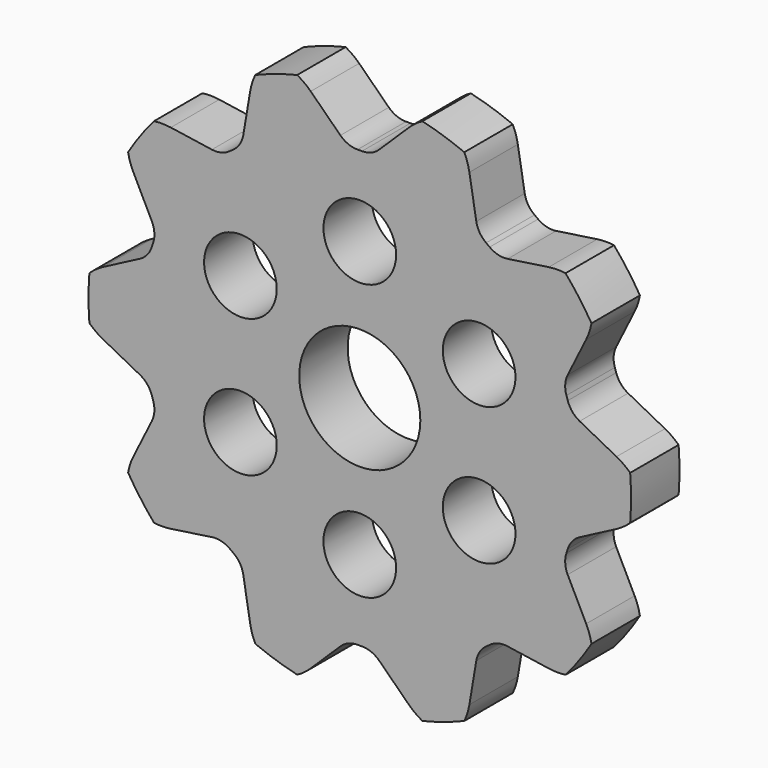
from build123d import *

# Parameters (mm, degrees)
F1_DEPTH        = 25
F3_DEPTH        = 25.001
F3_COPIES_COUNT = 10
F4_R            = 25
F5_DEPTH        = 25.001
F6_R            = 15
F7_DEPTH        = 25.001
F7_COPIES_COUNT = 6


# Not quite as in the source:
# - a pattern or mirror of a feature is missing from the dataset's text; its kind, count and spacing are read off the source's solid


with BuildPart() as f1:
    # F0 (on Front) → F1 (new body)
    with BuildSketch(Plane.XZ):
        with BuildLine():
            Line((-8.9100863455, 98.6570205686), (0, 100))
            Line((0, 100), (13.2558165823, 98.002007127))
            Line((13.2558165823, 98.002007127), (20.2559942473, 104.8591660301))
            ThreePointArc((20.2559942473, 104.8591660301), (22.9030212669, 107.1136465319), (25.8372403083, 108.979066858))
            ThreePointArc((25.8372403083, 108.979066858), (0, 112), (-25.8372403083, 108.979066858))
            ThreePointArc((-25.8372403083, 108.979066858), (-22.9030212669, 107.1136465319), (-20.2559942473, 104.8591660301))
            Line((-20.2559942473, 104.8591660301), (-13.2558165823, 98.002007127))
            Line((-13.2558165823, 98.002007127), (-8.9100863455, 98.6570205686))
        make_face()
        with BuildLine():
            Line((20.2559942473, 104.8591660301), (13.2558165823, 98.002007127))
            Line((13.2558165823, 98.002007127), (29.4755174411, 95.5572805786))
            Line((29.4755174411, 95.5572805786), (56.3320058064, 82.6238774316))
            Line((56.3320058064, 82.6238774316), (78.1831482468, 62.3489801859))
            Line((78.1831482468, 62.3489801859), (93.0873748644, 36.5341024366))
            Line((93.0873748644, 36.5341024366), (99.7203797181, 7.4730093586))
            Line((99.7203797181, 7.4730093586), (97.4927912182, -22.2520933956))
            Line((97.4927912182, -22.2520933956), (86.6025403784, -50))
            Line((86.6025403784, -50), (68.0172737771, -73.305187183))
            Line((68.0172737771, -73.305187183), (43.3883739118, -90.0968867902))
            Line((43.3883739118, -90.0968867902), (14.9042266176, -98.8830826225))
            Line((14.9042266176, -98.8830826225), (-14.9042266176, -98.8830826225))
            Line((-14.9042266176, -98.8830826225), (-43.3883739118, -90.0968867902))
            Line((-43.3883739118, -90.0968867902), (-68.0172737771, -73.305187183))
            Line((-68.0172737771, -73.305187183), (-86.6025403784, -50))
            Line((-86.6025403784, -50), (-97.4927912182, -22.2520933956))
            Line((-97.4927912182, -22.2520933956), (-99.7203797181, 7.4730093586))
            Line((-99.7203797181, 7.4730093586), (-93.0873748644, 36.5341024366))
            Line((-93.0873748644, 36.5341024366), (-78.1831482468, 62.3489801859))
            Line((-78.1831482468, 62.3489801859), (-56.3320058064, 82.6238774316))
            Line((-56.3320058064, 82.6238774316), (-29.4755174411, 95.5572805786))
            Line((-29.4755174411, 95.5572805786), (-13.2558165823, 98.002007127))
            Line((-13.2558165823, 98.002007127), (-20.2559942473, 104.8591660301))
            ThreePointArc((-20.2559942473, 104.8591660301), (-22.9030212669, 107.1136465319), (-25.8372403083, 108.979066858))
            ThreePointArc((-25.8372403083, 108.979066858), (-69.463044439, -87.857187852), (112, 0))
            ThreePointArc((112, 0), (87.857187852, 69.463044439), (25.8372403083, 108.979066858))
            ThreePointArc((25.8372403083, 108.979066858), (22.9030212669, 107.1136465319), (20.2559942473, 104.8591660301))
        make_face()
        with BuildLine():
            ThreePointArc((90, 0), (63.957016816, 63.3206127576), (0.9, 89.9954998875))
            ThreePointArc((0.9, 89.9954998875), (0, 90), (-0.9, 89.9954998875))
            ThreePointArc((-0.9, 89.9954998875), (-63.3206127576, -63.957016816), (90, 0))
        make_face()
        with BuildLine():
            Line((29.4755174411, 95.5572805786), (13.2558165823, 98.002007127))
            Line((13.2558165823, 98.002007127), (7.9977160698, 92.851333463))
            ThreePointArc((7.9977160698, 92.851333463), (4.7327694943, 90.7178003028), (0.9, 89.9954998875))
            ThreePointArc((0.9, 89.9954998875), (63.957016816, 63.3206127576), (90, 0))
            ThreePointArc((90, 0), (-63.3206127576, -63.957016816), (-0.9, 89.9954998875))
            ThreePointArc((-0.9, 89.9954998875), (-4.7327694943, 90.7178003028), (-7.9977160698, 92.851333463))
            Line((-7.9977160698, 92.851333463), (-13.2558165823, 98.002007127))
            Line((-13.2558165823, 98.002007127), (-29.4755174411, 95.5572805786))
            Line((-29.4755174411, 95.5572805786), (-56.3320058064, 82.6238774316))
            Line((-56.3320058064, 82.6238774316), (-78.1831482468, 62.3489801859))
            Line((-78.1831482468, 62.3489801859), (-93.0873748644, 36.5341024366))
            Line((-93.0873748644, 36.5341024366), (-99.7203797181, 7.4730093586))
            Line((-99.7203797181, 7.4730093586), (-97.4927912182, -22.2520933956))
            Line((-97.4927912182, -22.2520933956), (-86.6025403784, -50))
            Line((-86.6025403784, -50), (-68.0172737771, -73.305187183))
            Line((-68.0172737771, -73.305187183), (-43.3883739118, -90.0968867902))
            Line((-43.3883739118, -90.0968867902), (-14.9042266176, -98.8830826225))
            Line((-14.9042266176, -98.8830826225), (14.9042266176, -98.8830826225))
            Line((14.9042266176, -98.8830826225), (43.3883739118, -90.0968867902))
            Line((43.3883739118, -90.0968867902), (68.0172737771, -73.305187183))
            Line((68.0172737771, -73.305187183), (86.6025403784, -50))
            Line((86.6025403784, -50), (97.4927912182, -22.2520933956))
            Line((97.4927912182, -22.2520933956), (99.7203797181, 7.4730093586))
            Line((99.7203797181, 7.4730093586), (93.0873748644, 36.5341024366))
            Line((93.0873748644, 36.5341024366), (78.1831482468, 62.3489801859))
            Line((78.1831482468, 62.3489801859), (56.3320058064, 82.6238774316))
            Line((56.3320058064, 82.6238774316), (29.4755174411, 95.5572805786))
        make_face()
        with BuildLine():
            Line((13.2558165823, 98.002007127), (0, 100))
            Line((0, 100), (-8.9100863455, 98.6570205686))
            Line((-8.9100863455, 98.6570205686), (-13.2558165823, 98.002007127))
            Line((-13.2558165823, 98.002007127), (-7.9977160698, 92.851333463))
            ThreePointArc((-7.9977160698, 92.851333463), (-4.7327694943, 90.7178003028), (-0.9, 89.9954998875))
            ThreePointArc((-0.9, 89.9954998875), (0, 90), (0.9, 89.9954998875))
            ThreePointArc((0.9, 89.9954998875), (4.7327694943, 90.7178003028), (7.9977160698, 92.851333463))
            Line((7.9977160698, 92.851333463), (13.2558165823, 98.002007127))
        make_face()
    extrude(amount=F1_DEPTH)

    # F2 (on face) → F3 (cut, through all)
    with BuildSketch(Plane.XZ.offset(25)):
        with BuildLine():
            ThreePointArc((-25.8372403083, 108.979066858), (-22.9030212669, 107.1136465319), (-20.2559942473, 104.8591660301))
            Line((-20.2559942473, 104.8591660301), (-7.9977160698, 92.851333463))
            ThreePointArc((-7.9977160698, 92.851333463), (-4.7327694943, 90.7178003028), (-0.9, 89.9954998875))
            ThreePointArc((-0.9, 89.9954998875), (0, 90), (0.9, 89.9954998875))
            ThreePointArc((0.9, 89.9954998875), (4.7327694943, 90.7178003028), (7.9977160698, 92.851333463))
            Line((7.9977160698, 92.851333463), (20.2559942473, 104.8591660301))
            ThreePointArc((20.2559942473, 104.8591660301), (22.9030212669, 107.1136465319), (25.8372403083, 108.979066858))
            ThreePointArc((25.8372403083, 108.979066858), (0, 112), (-25.8372403083, 108.979066858))
        make_face()
    f3 = extrude(amount=-F3_DEPTH, mode=Mode.SUBTRACT)

    # F3_copies: F3 ×10 about axis
    f3_copies_axis = Axis((0, 0, 0), (0, 1, 0))
    for i in range(1, F3_COPIES_COUNT):
        add(f3.rotate(f3_copies_axis, i * 360 / F3_COPIES_COUNT), mode=Mode.SUBTRACT)

    # F4 (on face) → F5 (cut, through all)
    with BuildSketch(Plane.XZ.offset(25)):
        Circle(F4_R)
    extrude(amount=-F5_DEPTH, mode=Mode.SUBTRACT)

    # F6 (on face) → F7 (cut, through all)
    with BuildSketch(Plane.XZ.offset(25)):
        with Locations((0, 56.8999728613)):
            Circle(F6_R)
    f7 = extrude(amount=-F7_DEPTH, mode=Mode.SUBTRACT)

    # F7_copies: F7 ×6 about axis
    f7_copies_axis = Axis((0, 0, 0), (0, 1, 0))
    for i in range(1, F7_COPIES_COUNT):
        add(f7.rotate(f7_copies_axis, i * 360 / F7_COPIES_COUNT), mode=Mode.SUBTRACT)


solid = f1.part
